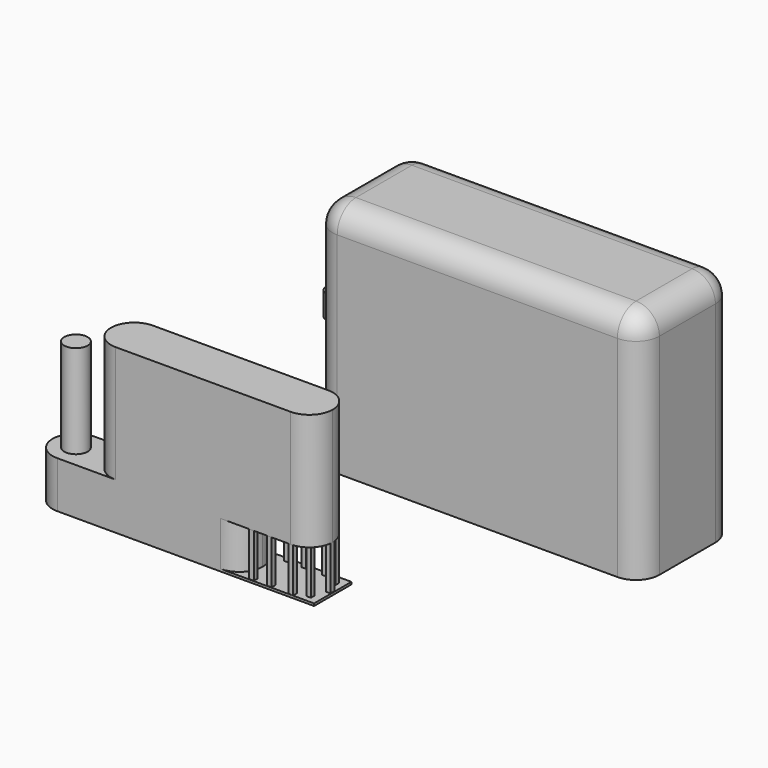
from build123d import *

# Parameters (mm, degrees)
F1_DEPTH  = 5
F0_R      = 7.5
F2_R      = 2.49999
F3_DEPTH  = 50
F4_W      = 50
F4_H      = 10
F5_DEPTH  = 20
F6_R      = 4.99999
F0_W      = 18.4688572213
F0_H      = 10
F0_W_2    = 41.5311427787
F7_DEPTH  = 10
F8_W      = 47.5
F8_H      = 10
F9_DEPTH  = 25
F10_W     = 10
F10_H     = 10
F11_DEPTH = 15
F12_R     = 3.5
F13_DEPTH = 20
F8_R      = 2.5
F14_DEPTH = 20
F15_R     = 4.99999
F16_W     = 1
F16_H     = 1
F17_DEPTH = 10
F18_DEPTH = 0.5


# Not quite as in the source:
# - a fillet or chamfer is up to 0.001 mm smaller than in the source, because OpenCascade refuses the exact size


with BuildPart() as f1:
    # F0 (on Top) → F1 (new body)
    with BuildSketch(Plane.XY):
        Polygon((-67.8614835593, 34.5565372526), (-67.8614835593, 29.5565372526), (-22.7404969164, 29.5565372526), (-28.6992648794, 34.5565372526), align=None)
        Polygon((-28.6992648794, 34.5565372526), (-22.7404969164, 29.5565372526), (-3.4568686258, 52.5378705461), (-9.4156365888, 57.5378705461), align=None)
    extrude(amount=F1_DEPTH)

    # F2 (radius 2.5 in the source; OpenCascade refuses exactly that, so slightly less here)
    f2_edges = [f1.edges().sort_by_distance(p)[0] for p in [
        (-28.699265, 34.556537, 2.5),
        (-67.861484, 34.556537, 2.5),
        (-67.861484, 29.556537, 2.5),
        (-22.740497, 29.556537, 2.5),
        (-3.456869, 52.537871, 2.5),
        (-9.415637, 57.537871, 2.5),
    ]]
    fillet(f2_edges, radius=F2_R)


with BuildPart() as f1b:
    # F0 (on Top) → F1, piece 2 (new body)
    with BuildSketch(Plane.XY):
        with Locations((4.2551979423, 17.4079854041)):
            Circle(F0_R)
    extrude(amount=F1_DEPTH)


with BuildPart() as f3:
    # F0 (on Top) → F3 (new body)
    with BuildSketch(Plane.XY):
        Polygon((-35, -12.5), (35, -12.5), (35, 12.5), (25, 12.5), (25, -7.5), (-25, -7.5), (-25, 12.5), (-35, 12.5), align=None)
    extrude(amount=F3_DEPTH)

    # F4 (on face) → F5 (join)
    with BuildSketch(Plane(origin=(0, -7.5, 0), x_dir=(-1, 0, 0), z_dir=(0, 1, 0))):
        with Locations((0, 45)):
            Rectangle(F4_W, F4_H)
    extrude(amount=F5_DEPTH)

    # F6 (radius 5 in the source; OpenCascade refuses exactly that, so slightly less here)
    f6_edges = [f3.edges().sort_by_distance(p)[0] for p in [
        (0, 12.5, 40),
        (25, 12.5, 20),
        (-25, 12.5, 20),
        (0, 12.5, 50),
        (35, 12.5, 25),
        (-35, 12.5, 25),
        (-35, 0, 50),
        (35, 0, 50),
        (0, -12.5, 50),
        (35, -12.5, 25),
        (-35, -12.5, 25),
    ]]
    fillet(f6_edges, radius=F6_R)


with BuildPart() as f7:
    # F0 (on Top) → F7 (new body)
    with BuildSketch(Plane.XY):
        with Locations((-53.8105743192, -47.3971840739)):
            Rectangle(F0_W, F0_H)
        with Locations((-23.8105743192, -47.3971840739)):
            Rectangle(F0_W_2, F0_H)
    extrude(amount=F7_DEPTH)

    # F8 (on face) → F9 (join)
    with BuildSketch(Plane.XY.offset(10)):
        with Locations((-26.7950029299, -47.3971840739)):
            Rectangle(F8_W, F8_H)
    extrude(amount=F9_DEPTH)

    # F10 (on face) → F11 (cut)
    with BuildSketch(Plane.YZ.offset(-3.0450029299)):
        with Locations((-47.3971840739, 5)):
            Rectangle(F10_W, F10_H)
    extrude(amount=-F11_DEPTH, mode=Mode.SUBTRACT)

    # F12 (on face) → F13 (cut)
    with BuildSketch(Plane(origin=(0, 0, 10), x_dir=(1, 0, 0), z_dir=(0, 0, -1))):
        with Locations((-8.0450029299, 47.3971840739)):
            Circle(F12_R)
    extrude(amount=-F13_DEPTH, mode=Mode.SUBTRACT)

    # F8 (on face) → F14 (join)
    with BuildSketch(Plane.XY.offset(10)):
        with Locations((-58.0450029299, -47.3971840739)):
            Circle(F8_R)
    extrude(amount=F14_DEPTH)

    # F15 (radius 5 in the source; OpenCascade refuses exactly that, so slightly less here)
    f15_edges = [f7.edges().sort_by_distance(p)[0] for p in [
        (-50.545003, -52.397184, 22.5),
        (-50.545003, -42.397184, 22.5),
        (-63.045003, -52.397184, 5),
        (-63.045003, -42.397184, 5),
        (-3.045003, -42.397184, 22.5),
        (-3.045003, -52.397184, 22.5),
        (-18.045003, -52.397184, 5),
        (-18.045003, -42.397184, 5),
    ]]
    fillet(f15_edges, radius=F15_R)

    # F16 (on face) → F17 (join)
    with BuildSketch(Plane(origin=(0, 0, 10), x_dir=(1, 0, 0), z_dir=(0, 0, -1))):
        with Locations((-16.5112521499, 51.7890639603)):
            Rectangle(F16_W, F16_H)
        with Locations((-12.7312513068, 51.7890639603)):
            Rectangle(F16_W, F16_H)
        with Locations((-8.0587519333, 51.8415607512)):
            Rectangle(F16_W, F16_H)
        with Locations((-5.2247602621, 50.6356314291)):
            Rectangle(F16_W, F16_H)
        with Locations((-3.6487516481, 47.3528131843)):
            Rectangle(F16_W, F16_H)
        with BuildLine():
            Line((-4.3825014383, 43.9933444551), (-4.3825014383, 44.9915629923))
            Line((-4.3825014383, 44.9915629923), (-5.3825014383, 44.9915629923))
            Line((-5.3825014383, 44.9915629923), (-5.3825014383, 43.9915629923))
            Line((-5.3825014383, 43.9915629923), (-4.3841578938, 43.9915629923))
            ThreePointArc((-4.3841578938, 43.9915629923), (-4.3833295577, 43.992453623), (-4.3825014383, 43.9933444551))
        make_face()
        with Locations((-7.9537518322, 42.9953113198)):
            Rectangle(F16_W, F16_H)
        with Locations((-12.388751924, 42.9703136086)):
            Rectangle(F16_W, F16_H)
        with Locations((-16.1175020039, 42.9953113198)):
            Rectangle(F16_W, F16_H)
    extrude(amount=F17_DEPTH)

    # F0 (on Top) → F18 (join)
    with BuildSketch(Plane.XY):
        with Locations((-23.8105743192, -47.3971840739)):
            Rectangle(F0_W_2, F0_H)
    extrude(amount=F18_DEPTH)


solid = Compound([f1.part, f1b.part, f3.part, f7.part])
